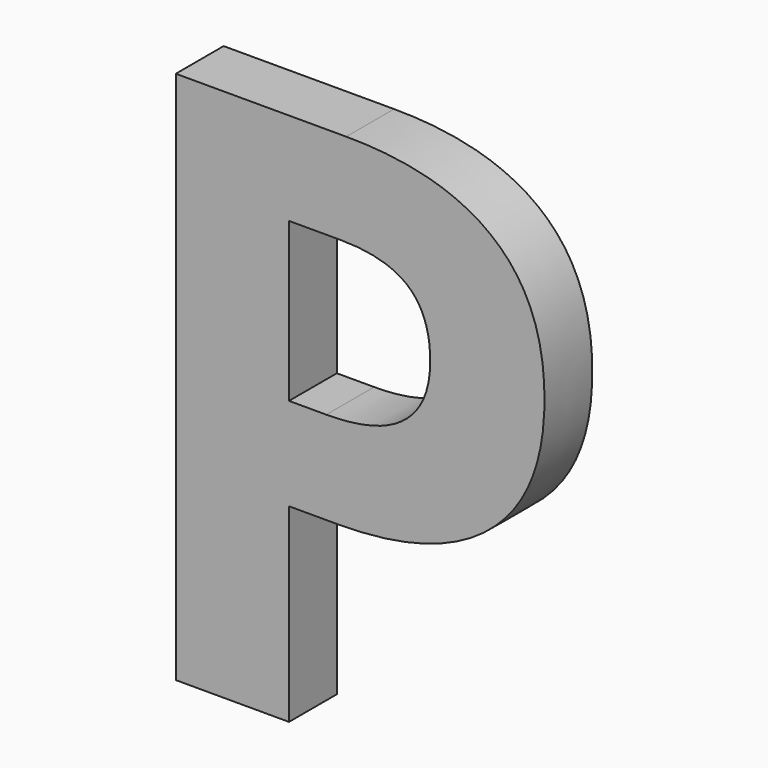
from build123d import *

# Parameters (mm, degrees)
F0_TEXT_SIZE = 62.5
F1_DEPTH     = 5


# Not quite as in the source:
# - Text() gives the source's letters only with a copy of the font that has no kerning and outlines rounded to 1/6400 em; it was checked with that copy


with BuildPart() as f1:
    # F0 (on Front) → F1 (new body)
    with BuildSketch(Plane.XZ):
        with Locations((-86.5348589579, 39.7540336407)):
            Text('P', F0_TEXT_SIZE, font='Open Sans', font_style=FontStyle.BOLD, text_align=(TextAlign.LEFT, TextAlign.BOTTOM))
    extrude(amount=F1_DEPTH)


solid = f1.part
